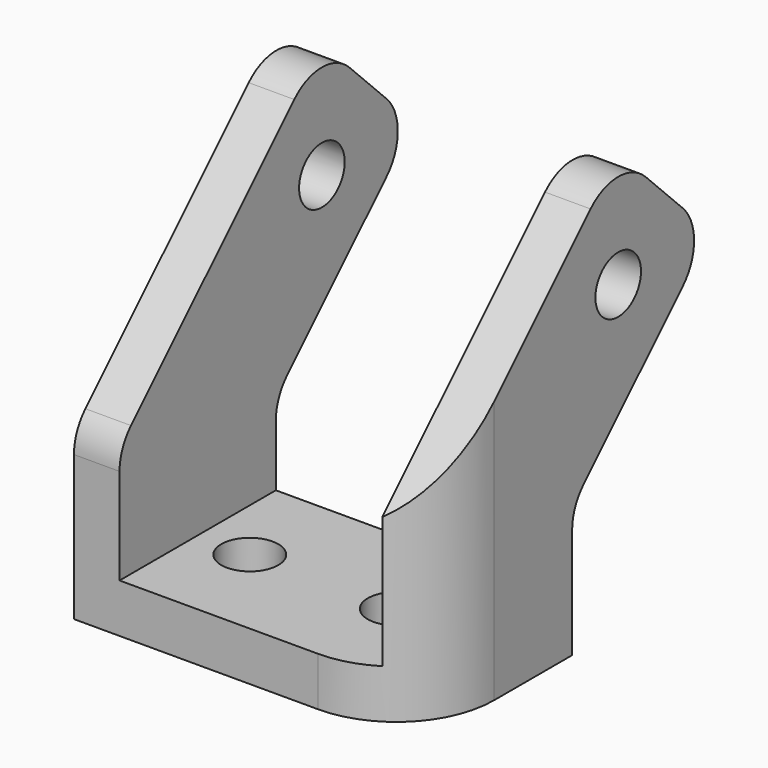
from build123d import *

# Parameters (mm, degrees)
F0_W        = 21
F0_H        = 12
F0_R        = 1.75
F1_DEPTH    = 3
F3_R        = 1.75
F4_DEPTH    = 2.8
F2_R        = 1.75
F5_DEPTH    = 2.8
F6_R        = 6
F7_T1_DEPTH = 2.8
F7_T3_DEPTH = 2.8
F7_T5_DEPTH = 17.8
F7_T7_DEPTH = 17.8
F7_T9_DEPTH = 9.0132034356


# Not quite as in the source:
# - a fillet or chamfer that OpenCascade refuses, or shapes differently, is made with other operations: its cross-section is extruded or revolved along the edge and cut away or added


with BuildPart() as f1:
    # F0 (on Top) → F1 (new body)
    with BuildSketch(Plane.XY):
        with Locations((10.5, 6)):
            Rectangle(F0_W, F0_H)
        with Locations((6, 6)):
            Circle(F0_R, mode=Mode.SUBTRACT)
        with Locations((15, 6)):
            Circle(F0_R, mode=Mode.SUBTRACT)
    extrude(amount=F1_DEPTH)

    # F3 (on face) → F4 (join)
    with BuildSketch(Plane.YZ.offset(21)):
        Polygon((0, 10.1421356237), (0, 3), (12, 3), (12, 8), (22.6066017178, 18.6066017178), (15.5355339059, 25.6776695297), align=None)
        with Locations((15.5355339059, 18.6066017178)):
            Circle(F3_R, mode=Mode.SUBTRACT)
    extrude(amount=-F4_DEPTH)

    # F2 (on face) → F5 (join)
    with BuildSketch(Plane(origin=(0, 0, 0), x_dir=(0, -1, 0), z_dir=(-1, 0, 0))):
        Polygon((-12, 8), (-12, 3), (0, 3), (0, 10.1421356237), (-15.5355339059, 25.6776695297), (-22.6066017178, 18.6066017178), align=None)
        with Locations((-15.5355339059, 18.6066017178)):
            Circle(F2_R, mode=Mode.SUBTRACT)
    extrude(amount=-F5_DEPTH)

    # F6
    f6_edges = [f1.edges().sort_by_distance(p)[0] for p in [
        (21, 0, 5.071068),
    ]]
    fillet(f6_edges, radius=F6_R)

    # F7: fillet of radius 3 on 8 edges, made by hand

    # F7_s2 → F7_t1 (join)
    with BuildSketch(Plane.YZ.offset(18.2)):
        with BuildLine():
            ThreePointArc((12, 6.7573593129), (12.2283614025, 7.90540961), (12.8786796564, 8.8786796564))
            Line((12.8786796564, 8.8786796564), (12, 8))
            Line((12, 8), (12, 6.7573593129))
        make_face()
    extrude(amount=F7_T1_DEPTH)

    # F7_s4 → F7_t3 (join)
    with BuildSketch(Plane.YZ):
        with BuildLine():
            ThreePointArc((12, 6.7573593129), (12.2283614025, 7.90540961), (12.8786796564, 8.8786796564))
            Line((12.8786796564, 8.8786796564), (12, 8))
            Line((12, 8), (12, 6.7573593129))
        make_face()
    extrude(amount=F7_T3_DEPTH)

    # F7_s6 → F7_t5 (cut)
    with BuildSketch(Plane.YZ.offset(-7.5)):
        with BuildLine():
            ThreePointArc((20.4852813742, 20.7279220614), (21.3639610307, 18.6066017178), (20.4852813742, 16.4852813742))
            Line((20.4852813742, 16.4852813742), (22.6066017178, 18.6066017178))
            Line((22.6066017178, 18.6066017178), (20.4852813742, 20.7279220614))
        make_face()
        with BuildLine():
            ThreePointArc((13.4142135624, 23.5563491861), (15.5355339059, 24.4350288425), (17.6568542495, 23.5563491861))
            Line((17.6568542495, 23.5563491861), (15.5355339059, 25.6776695297))
            Line((15.5355339059, 25.6776695297), (13.4142135624, 23.5563491861))
        make_face()
    extrude(amount=F7_T5_DEPTH, mode=Mode.SUBTRACT)

    # F7_s8 → F7_t7 (cut)
    with BuildSketch(Plane.YZ.offset(10.7)):
        with BuildLine():
            ThreePointArc((20.4852813742, 20.7279220614), (21.3639610307, 18.6066017178), (20.4852813742, 16.4852813742))
            Line((20.4852813742, 16.4852813742), (22.6066017178, 18.6066017178))
            Line((22.6066017178, 18.6066017178), (20.4852813742, 20.7279220614))
        make_face()
        with BuildLine():
            ThreePointArc((13.4142135624, 23.5563491861), (15.5355339059, 24.4350288425), (17.6568542495, 23.5563491861))
            Line((17.6568542495, 23.5563491861), (15.5355339059, 25.6776695297))
            Line((15.5355339059, 25.6776695297), (13.4142135624, 23.5563491861))
        make_face()
    extrude(amount=F7_T7_DEPTH, mode=Mode.SUBTRACT)

    # F7_s10 → F7_t9 (cut)
    with BuildSketch(Plane.YZ.offset(-3.1066017178)):
        with BuildLine():
            ThreePointArc((0, 8.8994949366), (0.2283614025, 10.0475452337), (0.8786796564, 11.0208152802))
            Line((0.8786796564, 11.0208152802), (0, 10.1421356237))
            Line((0, 10.1421356237), (0, 8.8994949366))
        make_face()
    extrude(amount=F7_T9_DEPTH, mode=Mode.SUBTRACT)


solid = f1.part
